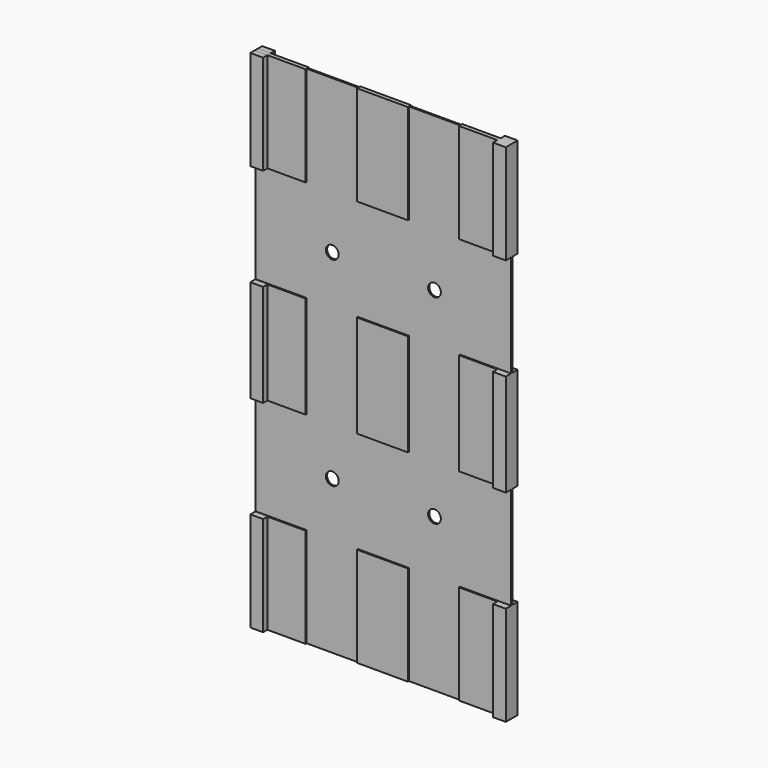
from build123d import *

# Parameters (mm, degrees)
F0_W     = 5
F0_H     = 39
F1_DEPTH = 2.9
F0_H_2   = 40
F0_W_2   = 15
F2_DEPTH = 0.8
F0_W_3   = 20
F3_DEPTH = 0.3
F4_R     = 2.5
F5_DEPTH = 3.201


with BuildPart() as f1:
    # F0 (on Front) → F1 (new body, symmetric)
    with BuildSketch(Plane.XZ):
        with Locations((-47.5, -79.5)):
            Rectangle(F0_W, F0_H)
    extrude(amount=F1_DEPTH, both=True)


with BuildPart() as f1b:
    # F0 (on Front) → F1, piece 2 (new body, symmetric)
    with BuildSketch(Plane.XZ):
        with Locations((-47.5, 79.5)):
            Rectangle(F0_W, F0_H)
    extrude(amount=F1_DEPTH, both=True)


with BuildPart() as f1c:
    # F0 (on Front) → F1, piece 3 (new body, symmetric)
    with BuildSketch(Plane.XZ):
        with Locations((-47.5, 0)):
            Rectangle(F0_W, F0_H_2)
    extrude(amount=F1_DEPTH, both=True)


with BuildPart() as f1d:
    # F0 (on Front) → F1, piece 4 (new body, symmetric)
    with BuildSketch(Plane.XZ):
        with Locations((47.5, -79.5)):
            Rectangle(F0_W, F0_H)
    extrude(amount=F1_DEPTH, both=True)

    # F0 (on Front) → F2, piece 4 (join, symmetric)
    with BuildSketch(Plane.XZ):
        with Locations((37.5, -79.5)):
            Rectangle(F0_W_2, F0_H)
    extrude(amount=F2_DEPTH, both=True)


with BuildPart() as f1e:
    # F0 (on Front) → F1, piece 5 (new body, symmetric)
    with BuildSketch(Plane.XZ):
        with Locations((47.5, 79.5)):
            Rectangle(F0_W, F0_H)
    extrude(amount=F1_DEPTH, both=True)

    # F0 (on Front) → F2, piece 5 (join, symmetric)
    with BuildSketch(Plane.XZ):
        with Locations((37.5, 79.5)):
            Rectangle(F0_W_2, F0_H)
    extrude(amount=F2_DEPTH, both=True)


with BuildPart() as f1f:
    # F0 (on Front) → F1, piece 6 (new body, symmetric)
    with BuildSketch(Plane.XZ):
        with Locations((47.5, 0)):
            Rectangle(F0_W, F0_H_2)
    extrude(amount=F1_DEPTH, both=True)


with BuildPart() as f2:
    # F0 (on Front) → F2 (new body, symmetric)
    with BuildSketch(Plane.XZ):
        with Locations((-37.5, -79.5)):
            Rectangle(F0_W_2, F0_H)
        with Locations((-47.5, -79.5)):
            Rectangle(F0_W, F0_H)
    extrude(amount=F2_DEPTH, both=True)


with BuildPart() as f2b:
    # F0 (on Front) → F2, piece 2 (new body, symmetric)
    with BuildSketch(Plane.XZ):
        with Locations((-37.5, 79.5)):
            Rectangle(F0_W_2, F0_H)
        with Locations((-47.5, 79.5)):
            Rectangle(F0_W, F0_H)
    extrude(amount=F2_DEPTH, both=True)


with BuildPart() as f2c:
    # F0 (on Front) → F2, piece 3 (new body, symmetric)
    with BuildSketch(Plane.XZ):
        with Locations((-37.5, 0)):
            Rectangle(F0_W_2, F0_H_2)
        with Locations((-47.5, 0)):
            Rectangle(F0_W, F0_H_2)
    extrude(amount=F2_DEPTH, both=True)


with BuildPart() as f2d:
    # F0 (on Front) → F2, piece 6 (new body, symmetric)
    with BuildSketch(Plane.XZ):
        with Locations((37.5, 0)):
            Rectangle(F0_W_2, F0_H_2)
    extrude(amount=F2_DEPTH, both=True)


with BuildPart() as f2e:
    # F0 (on Front) → F2, piece 7 (new body, symmetric)
    with BuildSketch(Plane.XZ):
        with Locations((0, -79.5)):
            Rectangle(F0_W_3, F0_H)
    extrude(amount=F2_DEPTH, both=True)


with BuildPart() as f2f:
    # F0 (on Front) → F2, piece 8 (new body, symmetric)
    with BuildSketch(Plane.XZ):
        with Locations((0, 79.5)):
            Rectangle(F0_W_3, F0_H)
    extrude(amount=F2_DEPTH, both=True)


with BuildPart() as f2g:
    # F0 (on Front) → F2, piece 9 (new body, symmetric)
    with BuildSketch(Plane.XZ):
        Rectangle(F0_W_3, F0_H_2)
    extrude(amount=F2_DEPTH, both=True)


with BuildPart() as f3:
    # F0 (on Front) → F3 (new body, symmetric)
    with BuildSketch(Plane.XZ):
        with Locations((-20, 79.5)):
            Rectangle(F0_W_3, F0_H)
        with Locations((-20, 40)):
            Rectangle(F0_W_3, F0_H_2)
        with Locations((-20, 0)):
            Rectangle(F0_W_3, F0_H_2)
        with Locations((-20, -40)):
            Rectangle(F0_W_3, F0_H_2)
        with Locations((-20, -79.5)):
            Rectangle(F0_W_3, F0_H)
        with Locations((20, 79.5)):
            Rectangle(F0_W_3, F0_H)
        with Locations((20, 40)):
            Rectangle(F0_W_3, F0_H_2)
        with Locations((20, 0)):
            Rectangle(F0_W_3, F0_H_2)
        with Locations((20, -40)):
            Rectangle(F0_W_3, F0_H_2)
        with Locations((20, -79.5)):
            Rectangle(F0_W_3, F0_H)
        with Locations((-47.5, 40)):
            Rectangle(F0_W, F0_H_2)
        with Locations((-37.5, 40)):
            Rectangle(F0_W_2, F0_H_2)
        with Locations((0, 40)):
            Rectangle(F0_W_3, F0_H_2)
        with Locations((37.5, 40)):
            Rectangle(F0_W_2, F0_H_2)
        with Locations((47.5, 40)):
            Rectangle(F0_W, F0_H_2)
        with Locations((47.5, -40)):
            Rectangle(F0_W, F0_H_2)
        with Locations((37.5, -40)):
            Rectangle(F0_W_2, F0_H_2)
        with Locations((0, -40)):
            Rectangle(F0_W_3, F0_H_2)
        with Locations((-37.5, -40)):
            Rectangle(F0_W_2, F0_H_2)
        with Locations((-47.5, -40)):
            Rectangle(F0_W, F0_H_2)
    extrude(amount=F3_DEPTH, both=True)

    # F4 (on face) → F5 (cut, through all)
    with BuildSketch(Plane.XZ.offset(0.3)):
        with Locations((-20, 39)):
            Circle(F4_R)
        with Locations((20, 39)):
            Circle(F4_R)
        with Locations((-20, -39)):
            Circle(F4_R)
        with Locations((20, -39)):
            Circle(F4_R)
    extrude(amount=-F5_DEPTH, mode=Mode.SUBTRACT)


solid = Compound([f1.part, f1b.part, f1c.part, f1d.part, f1e.part, f1f.part, f2.part, f2b.part, f2c.part, f2d.part, f2e.part, f2f.part, f2g.part, f3.part])
